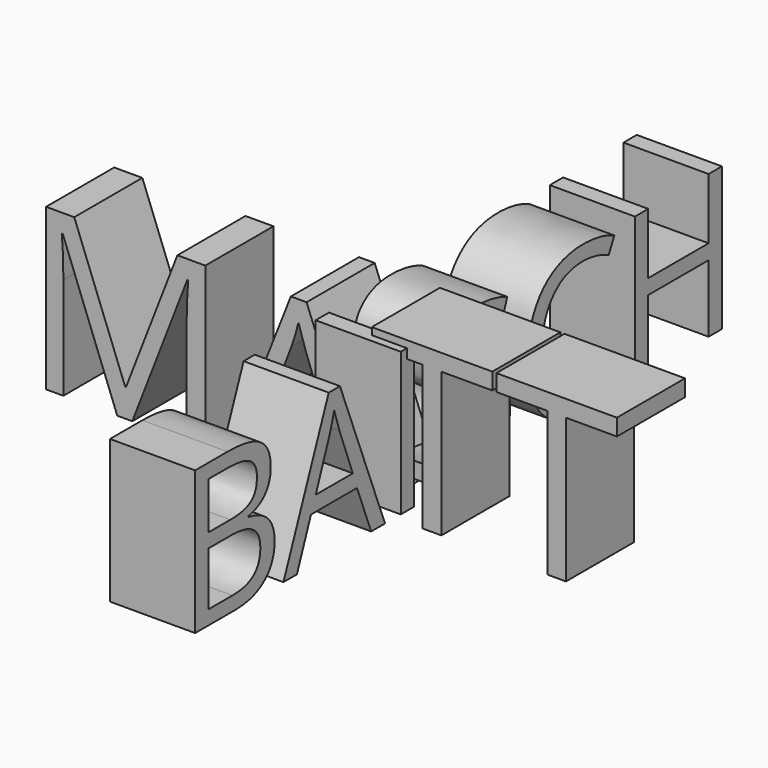
from build123d import *

# Parameters (mm, degrees)
F1_TEXT_SIZE = 59.869670723
F2_DEPTH     = 25.4
F0_TEXT_SIZE = 67.191860742
F3_DEPTH     = 25.4


# Not quite as in the source:
# - Text() gives the source's letters only with a copy of the font that has no kerning and outlines rounded to 1/6400 em; it was checked with that copy


with BuildPart() as f2:
    # F1 (on Right) → F2 (new body)
    with BuildSketch(Plane.YZ):
        with Locations((-110.2463379502, -20.9328494966)):
            Text('BAISCH', F1_TEXT_SIZE, font='Open Sans', text_align=(TextAlign.LEFT, TextAlign.BOTTOM))
    extrude(amount=F2_DEPTH)


with BuildPart() as f3:
    # F0 (on Front) → F3 (new body)
    with BuildSketch(Plane.XZ):
        with Locations((-88.8483226299, -24.034012109)):
            Text('MATT', F0_TEXT_SIZE, font='Open Sans', text_align=(TextAlign.LEFT, TextAlign.BOTTOM))
    extrude(amount=F3_DEPTH)


solid = Compound([f2.part, f3.part])
